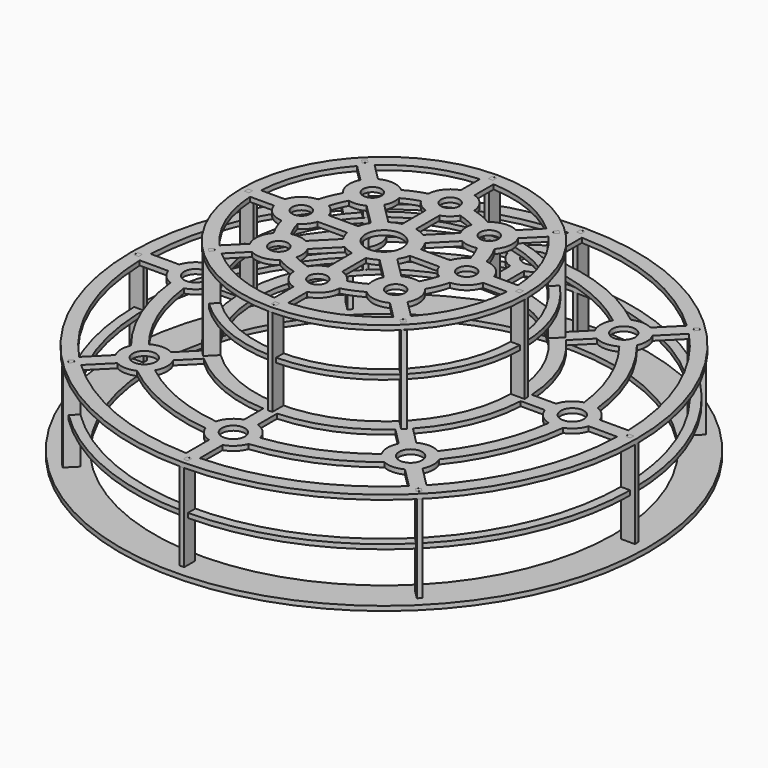
from build123d import *

# Parameters (mm, degrees)
F4_R      = 550
F4_R_2    = 25
F4_R_3    = 280
F5_DEPTH  = 10
F6_R      = 310
F6_R_2    = 20
F6_R_3    = 40
F7_DEPTH  = 10
F8_R      = 575
F8_R_2    = 500
F9_DEPTH  = 10
F11_DEPTH = 5
F12_COUNT = 8
F13_R     = 520
F14_DEPTH = 10
F15_R     = 280
F16_DEPTH = 10


with BuildPart() as f5:
    # F4 (on Top) → F5 (new body)
    with BuildSketch(Plane.XY):
        Circle(F4_R)
        Polygon((-374.0594872477, -375.4737008101), (-371.3017708011, -378.2314172567), (-378.3728386129, -385.3024850685), (-381.1305550595, -382.5447686219), (-382.5447686219, -382.5447686219), (-382.5447686219, -381.1305550595), (-385.3024850685, -378.3728386129), (-378.2314172567, -371.3017708011), (-375.4737008101, -374.0594872477), (-374.0594872477, -374.0594872477), align=None, mode=Mode.SUBTRACT)
        with Locations((-289.9137802865, -289.9137802865)):
            Circle(F4_R_2, mode=Mode.SUBTRACT)
        with BuildLine():
            ThreePointArc((-46.8602222393, -427.4390243902), (-34.4319247471, -446.2552418033), (-15, -457.6969600708))
            Line((-15, -457.6969600708), (-15, -519.783608822))
            ThreePointArc((-15, -519.783608822), (-198.9953848298, -480.4173569059), (-356.9359128298, -378.1491162654))
            Line((-356.9359128298, -378.1491162654), (-313.0340224768, -334.2472259124))
            ThreePointArc((-313.0340224768, -334.2472259124), (-291.2030601412, -339.8971550971), (-269.1098517768, -335.3802136034))
            ThreePointArc((-269.1098517768, -335.3802136034), (-164.553875917, -397.2681989799), (-46.8602222393, -427.4390243902))
        make_face(mode=Mode.SUBTRACT)
        with BuildLine():
            Line((-15, -309.6368841078), (-15, -362.3030399292))
            ThreePointArc((-15, -362.3030399292), (-36.1104599854, -375.4162656782), (-48.3000733443, -397.0731707317))
            ThreePointArc((-48.3000733443, -397.0731707317), (-153.073372946, -369.5518130045), (-246.619822258, -314.9264410452))
            ThreePointArc((-246.619822258, -314.9264410452), (-239.9254361013, -290.9933383562), (-245.5803346606, -266.7935380962))
            Line((-245.5803346606, -266.7935380962), (-208.3397387403, -229.5529421759))
            ThreePointArc((-208.3397387403, -229.5529421759), (-118.6318640332, -286.4026550785), (-15, -309.6368841078))
        make_face(mode=Mode.SUBTRACT)
        with BuildLine():
            Line((-519.783608822, -15), (-457.6969600708, -15))
            ThreePointArc((-457.6969600708, -15), (-446.2552418033, -34.4319247471), (-427.4390243902, -46.8602222393))
            ThreePointArc((-427.4390243902, -46.8602222393), (-397.2681989799, -164.553875917), (-335.3802136034, -269.1098517768))
            ThreePointArc((-335.3802136034, -269.1098517768), (-339.8971550971, -291.2030601412), (-334.2472259124, -313.0340224768))
            Line((-334.2472259124, -313.0340224768), (-378.1491162654, -356.9359128298))
            ThreePointArc((-378.1491162654, -356.9359128298), (-480.4173569059, -198.9953848298), (-519.783608822, -15))
        make_face(mode=Mode.SUBTRACT)
        with BuildLine():
            ThreePointArc((-397.0731707317, -48.3000733443), (-375.4162656782, -36.1104599854), (-362.3030399292, -15))
            Line((-362.3030399292, -15), (-309.6368841078, -15))
            ThreePointArc((-309.6368841078, -15), (-286.4026550785, -118.6318640332), (-229.5529421759, -208.3397387403))
            Line((-229.5529421759, -208.3397387403), (-266.7935380962, -245.5803346606))
            ThreePointArc((-266.7935380962, -245.5803346606), (-290.9933383562, -239.9254361013), (-314.9264410452, -246.619822258))
            ThreePointArc((-314.9264410452, -246.619822258), (-369.5518130045, -153.073372946), (-397.0731707317, -48.3000733443))
        make_face(mode=Mode.SUBTRACT)
        Polygon((-215.5968575838, -208.6672111282), (-208.5257897719, -201.5961433163), (-205.7680733253, -204.3538597629), (-204.3538597629, -204.3538597629), (-204.3538597629, -205.7680733253), (-201.5961433163, -208.5257897719), (-208.6672111282, -215.5968575838), (-211.4249275748, -212.8391411372), (-212.8391411372, -212.8391411372), (-212.8391411372, -211.4249275748), align=None, mode=Mode.SUBTRACT)
        Polygon((1, -530), (4.9, -530), (4.9, -540), (1, -540), (0, -541), (-1, -540), (-4.9, -540), (-4.9, -530), (-1, -530), (0, -529), align=None, mode=Mode.SUBTRACT)
        with BuildLine():
            ThreePointArc((356.9359128298, -378.1491162654), (198.9953848298, -480.4173569059), (15, -519.783608822))
            Line((15, -519.783608822), (15, -457.6969600708))
            ThreePointArc((15, -457.6969600708), (34.4319247471, -446.2552418033), (46.8602222393, -427.4390243902))
            ThreePointArc((46.8602222393, -427.4390243902), (164.553875917, -397.2681989799), (269.1098517768, -335.3802136034))
            ThreePointArc((269.1098517768, -335.3802136034), (291.2030601412, -339.8971550971), (313.0340224768, -334.2472259124))
            Line((313.0340224768, -334.2472259124), (356.9359128298, -378.1491162654))
        make_face(mode=Mode.SUBTRACT)
        with Locations((0, -410)):
            Circle(F4_R_2, mode=Mode.SUBTRACT)
        Polygon((-4.9, -300), (-4.9, -290), (-1, -290), (0, -289), (1, -290), (4.9, -290), (4.9, -300), (1, -300), (0, -301), (-1, -300), align=None, mode=Mode.SUBTRACT)
        with BuildLine():
            ThreePointArc((246.619822258, -314.9264410452), (153.073372946, -369.5518130045), (48.3000733443, -397.0731707317))
            ThreePointArc((48.3000733443, -397.0731707317), (36.1104599854, -375.4162656782), (15, -362.3030399292))
            Line((15, -362.3030399292), (15, -309.6368841078))
            ThreePointArc((15, -309.6368841078), (118.6318640332, -286.4026550785), (208.3397387403, -229.5529421759))
            Line((208.3397387403, -229.5529421759), (245.5803346606, -266.7935380962))
            ThreePointArc((245.5803346606, -266.7935380962), (239.9254361013, -290.9933383562), (246.619822258, -314.9264410452))
        make_face(mode=Mode.SUBTRACT)
        Polygon((375.4737008101, -374.0594872477), (378.2314172567, -371.3017708011), (385.3024850685, -378.3728386129), (382.5447686219, -381.1305550595), (382.5447686219, -382.5447686219), (381.1305550595, -382.5447686219), (378.3728386129, -385.3024850685), (371.3017708011, -378.2314172567), (374.0594872477, -375.4737008101), (374.0594872477, -374.0594872477), align=None, mode=Mode.SUBTRACT)
        with Locations((289.9137802865, -289.9137802865)):
            Circle(F4_R_2, mode=Mode.SUBTRACT)
        Polygon((208.6672111282, -215.5968575838), (201.5961433163, -208.5257897719), (204.3538597629, -205.7680733253), (204.3538597629, -204.3538597629), (205.7680733253, -204.3538597629), (208.5257897719, -201.5961433163), (215.5968575838, -208.6672111282), (212.8391411372, -211.4249275748), (212.8391411372, -212.8391411372), (211.4249275748, -212.8391411372), align=None, mode=Mode.SUBTRACT)
        with BuildLine():
            Line((378.1491162654, -356.9359128298), (334.2472259124, -313.0340224768))
            ThreePointArc((334.2472259124, -313.0340224768), (339.8971550971, -291.2030601412), (335.3802136034, -269.1098517768))
            ThreePointArc((335.3802136034, -269.1098517768), (397.2681989799, -164.553875917), (427.4390243902, -46.8602222393))
            ThreePointArc((427.4390243902, -46.8602222393), (446.2552418033, -34.4319247471), (457.6969600708, -15))
            Line((457.6969600708, -15), (519.783608822, -15))
            ThreePointArc((519.783608822, -15), (480.4173569059, -198.9953848298), (378.1491162654, -356.9359128298))
        make_face(mode=Mode.SUBTRACT)
        with BuildLine():
            ThreePointArc((314.9264410452, -246.619822258), (290.9933383562, -239.9254361013), (266.7935380962, -245.5803346606))
            Line((266.7935380962, -245.5803346606), (229.5529421759, -208.3397387403))
            ThreePointArc((229.5529421759, -208.3397387403), (286.4026550785, -118.6318640332), (309.6368841078, -15))
            Line((309.6368841078, -15), (362.3030399292, -15))
            ThreePointArc((362.3030399292, -15), (375.4162656782, -36.1104599854), (397.0731707317, -48.3000733443))
            ThreePointArc((397.0731707317, -48.3000733443), (369.5518130045, -153.073372946), (314.9264410452, -246.619822258))
        make_face(mode=Mode.SUBTRACT)
        Polygon((-530, -1), (-530, -4.9), (-540, -4.9), (-540, -1), (-541, 0), (-540, 1), (-540, 4.9), (-530, 4.9), (-530, 1), (-529, 0), align=None, mode=Mode.SUBTRACT)
        with Locations((-410, 0)):
            Circle(F4_R_2, mode=Mode.SUBTRACT)
        Polygon((-300, 4.9), (-290, 4.9), (-290, 1), (-289, 0), (-290, -1), (-290, -4.9), (-300, -4.9), (-300, -1), (-301, 0), (-300, 1), align=None, mode=Mode.SUBTRACT)
        with BuildLine():
            ThreePointArc((-314.9264410452, 246.619822258), (-290.9933383562, 239.9254361013), (-266.7935380962, 245.5803346606))
            Line((-266.7935380962, 245.5803346606), (-229.5529421759, 208.3397387403))
            ThreePointArc((-229.5529421759, 208.3397387403), (-286.4026550785, 118.6318640332), (-309.6368841078, 15))
            Line((-309.6368841078, 15), (-362.3030399292, 15))
            ThreePointArc((-362.3030399292, 15), (-375.4162656782, 36.1104599854), (-397.0731707317, 48.3000733443))
            ThreePointArc((-397.0731707317, 48.3000733443), (-369.5518130045, 153.073372946), (-314.9264410452, 246.619822258))
        make_face(mode=Mode.SUBTRACT)
        with BuildLine():
            Line((-378.1491162654, 356.9359128298), (-334.2472259124, 313.0340224768))
            ThreePointArc((-334.2472259124, 313.0340224768), (-339.8971550971, 291.2030601412), (-335.3802136034, 269.1098517768))
            ThreePointArc((-335.3802136034, 269.1098517768), (-397.2681989799, 164.553875917), (-427.4390243902, 46.8602222393))
            ThreePointArc((-427.4390243902, 46.8602222393), (-446.2552418033, 34.4319247471), (-457.6969600708, 15))
            Line((-457.6969600708, 15), (-519.783608822, 15))
            ThreePointArc((-519.783608822, 15), (-480.4173569059, 198.9953848298), (-378.1491162654, 356.9359128298))
        make_face(mode=Mode.SUBTRACT)
        Polygon((-208.6672111282, 215.5968575838), (-201.5961433163, 208.5257897719), (-204.3538597629, 205.7680733253), (-204.3538597629, 204.3538597629), (-205.7680733253, 204.3538597629), (-208.5257897719, 201.5961433163), (-215.5968575838, 208.6672111282), (-212.8391411372, 211.4249275748), (-212.8391411372, 212.8391411372), (-211.4249275748, 212.8391411372), align=None, mode=Mode.SUBTRACT)
        with Locations((-289.9137802865, 289.9137802865)):
            Circle(F4_R_2, mode=Mode.SUBTRACT)
        Polygon((-375.4737008101, 374.0594872477), (-378.2314172567, 371.3017708011), (-385.3024850685, 378.3728386129), (-382.5447686219, 381.1305550595), (-382.5447686219, 382.5447686219), (-381.1305550595, 382.5447686219), (-378.3728386129, 385.3024850685), (-371.3017708011, 378.2314172567), (-374.0594872477, 375.4737008101), (-374.0594872477, 374.0594872477), align=None, mode=Mode.SUBTRACT)
        with BuildLine():
            ThreePointArc((-48.3000733443, 397.0731707317), (-36.1104599854, 375.4162656782), (-15, 362.3030399292))
            Line((-15, 362.3030399292), (-15, 309.6368841078))
            ThreePointArc((-15, 309.6368841078), (-118.6318640332, 286.4026550785), (-208.3397387403, 229.5529421759))
            Line((-208.3397387403, 229.5529421759), (-245.5803346606, 266.7935380962))
            ThreePointArc((-245.5803346606, 266.7935380962), (-239.9254361013, 290.9933383562), (-246.619822258, 314.9264410452))
            ThreePointArc((-246.619822258, 314.9264410452), (-153.073372946, 369.5518130045), (-48.3000733443, 397.0731707317))
        make_face(mode=Mode.SUBTRACT)
        with BuildLine():
            Line((-15, 519.783608822), (-15, 457.6969600708))
            ThreePointArc((-15, 457.6969600708), (-34.4319247471, 446.2552418033), (-46.8602222393, 427.4390243902))
            ThreePointArc((-46.8602222393, 427.4390243902), (-164.553875917, 397.2681989799), (-269.1098517768, 335.3802136034))
            ThreePointArc((-269.1098517768, 335.3802136034), (-291.2030601412, 339.8971550971), (-313.0340224768, 334.2472259124))
            Line((-313.0340224768, 334.2472259124), (-356.9359128298, 378.1491162654))
            ThreePointArc((-356.9359128298, 378.1491162654), (-198.9953848298, 480.4173569059), (-15, 519.783608822))
        make_face(mode=Mode.SUBTRACT)
        Circle(F4_R_3, mode=Mode.SUBTRACT)
        Polygon((215.5968575838, 208.6672111282), (208.5257897719, 201.5961433163), (205.7680733253, 204.3538597629), (204.3538597629, 204.3538597629), (204.3538597629, 205.7680733253), (201.5961433163, 208.5257897719), (208.6672111282, 215.5968575838), (211.4249275748, 212.8391411372), (212.8391411372, 212.8391411372), (212.8391411372, 211.4249275748), align=None, mode=Mode.SUBTRACT)
        Polygon((300, -4.9), (290, -4.9), (290, -1), (289, 0), (290, 1), (290, 4.9), (300, 4.9), (300, 1), (301, 0), (300, -1), align=None, mode=Mode.SUBTRACT)
        with Locations((410, 0)):
            Circle(F4_R_2, mode=Mode.SUBTRACT)
        with BuildLine():
            ThreePointArc((397.0731707317, 48.3000733443), (375.4162656782, 36.1104599854), (362.3030399292, 15))
            Line((362.3030399292, 15), (309.6368841078, 15))
            ThreePointArc((309.6368841078, 15), (286.4026550785, 118.6318640332), (229.5529421759, 208.3397387403))
            Line((229.5529421759, 208.3397387403), (266.7935380962, 245.5803346606))
            ThreePointArc((266.7935380962, 245.5803346606), (290.9933383562, 239.9254361013), (314.9264410452, 246.619822258))
            ThreePointArc((314.9264410452, 246.619822258), (369.5518130045, 153.073372946), (397.0731707317, 48.3000733443))
        make_face(mode=Mode.SUBTRACT)
        Polygon((530, 1), (530, 4.9), (540, 4.9), (540, 1), (541, 0), (540, -1), (540, -4.9), (530, -4.9), (530, -1), (529, 0), align=None, mode=Mode.SUBTRACT)
        with BuildLine():
            Line((519.783608822, 15), (457.6969600708, 15))
            ThreePointArc((457.6969600708, 15), (446.2552418033, 34.4319247471), (427.4390243902, 46.8602222393))
            ThreePointArc((427.4390243902, 46.8602222393), (397.2681989799, 164.553875917), (335.3802136034, 269.1098517768))
            ThreePointArc((335.3802136034, 269.1098517768), (339.8971550971, 291.2030601412), (334.2472259124, 313.0340224768))
            Line((334.2472259124, 313.0340224768), (378.1491162654, 356.9359128298))
            ThreePointArc((378.1491162654, 356.9359128298), (480.4173569059, 198.9953848298), (519.783608822, 15))
        make_face(mode=Mode.SUBTRACT)
        Polygon((4.9, 300), (4.9, 290), (1, 290), (0, 289), (-1, 290), (-4.9, 290), (-4.9, 300), (-1, 300), (0, 301), (1, 300), align=None, mode=Mode.SUBTRACT)
        with BuildLine():
            ThreePointArc((246.619822258, 314.9264410452), (239.9254361013, 290.9933383562), (245.5803346606, 266.7935380962))
            Line((245.5803346606, 266.7935380962), (208.3397387403, 229.5529421759))
            ThreePointArc((208.3397387403, 229.5529421759), (118.6318640332, 286.4026550785), (15, 309.6368841078))
            Line((15, 309.6368841078), (15, 362.3030399292))
            ThreePointArc((15, 362.3030399292), (36.1104599854, 375.4162656782), (48.3000733443, 397.0731707317))
            ThreePointArc((48.3000733443, 397.0731707317), (153.073372946, 369.5518130045), (246.619822258, 314.9264410452))
        make_face(mode=Mode.SUBTRACT)
        with Locations((0, 410)):
            Circle(F4_R_2, mode=Mode.SUBTRACT)
        Polygon((4.9, 540), (4.9, 530), (1, 530), (0, 529), (-1, 530), (-4.9, 530), (-4.9, 540), (-1, 540), (0, 541), (1, 540), align=None, mode=Mode.SUBTRACT)
        with BuildLine():
            Line((356.9359128298, 378.1491162654), (313.0340224768, 334.2472259124))
            ThreePointArc((313.0340224768, 334.2472259124), (291.2030601412, 339.8971550971), (269.1098517768, 335.3802136034))
            ThreePointArc((269.1098517768, 335.3802136034), (164.553875917, 397.2681989799), (46.8602222393, 427.4390243902))
            ThreePointArc((46.8602222393, 427.4390243902), (34.4319247471, 446.2552418033), (15, 457.6969600708))
            Line((15, 457.6969600708), (15, 519.783608822))
            ThreePointArc((15, 519.783608822), (198.9953848298, 480.4173569059), (356.9359128298, 378.1491162654))
        make_face(mode=Mode.SUBTRACT)
        with Locations((289.9137802865, 289.9137802865)):
            Circle(F4_R_2, mode=Mode.SUBTRACT)
        Polygon((374.0594872477, 375.4737008101), (371.3017708011, 378.2314172567), (378.3728386129, 385.3024850685), (381.1305550595, 382.5447686219), (382.5447686219, 382.5447686219), (382.5447686219, 381.1305550595), (385.3024850685, 378.3728386129), (378.2314172567, 371.3017708011), (375.4737008101, 374.0594872477), (374.0594872477, 374.0594872477), align=None, mode=Mode.SUBTRACT)
    extrude(amount=F5_DEPTH)


with BuildPart() as f7:
    # F6 (on offset) → F7 (new body)
    with BuildSketch(Plane.XY.offset(200)):
        Circle(F6_R)
        Polygon((-204.3538597629, -204.3538597629), (-204.3538597629, -205.7680733253), (-201.5961433163, -208.5257897719), (-208.6672111282, -215.5968575838), (-211.4249275748, -212.8391411372), (-212.8391411372, -212.8391411372), (-212.8391411372, -211.4249275748), (-215.5968575838, -208.6672111282), (-208.5257897719, -201.5961433163), (-205.7680733253, -204.3538597629), align=None, mode=Mode.SUBTRACT)
        with BuildLine():
            ThreePointArc((-49.888765157, -183.3333333333), (-39.3023002536, -210.9084000682), (-15, -227.6969600708))
            Line((-15, -227.6969600708), (-15, -279.5979256003))
            ThreePointArc((-15, -279.5979256003), (-107.1513610622, -258.6862691032), (-187.0989874799, -208.3121909155))
            Line((-187.0989874799, -208.3121909155), (-150.3994628039, -171.6126662395))
            ThreePointArc((-150.3994628039, -171.6126662395), (-121.3438368718, -176.925682923), (-94.35955907, -164.9129273651))
            ThreePointArc((-94.35955907, -164.9129273651), (-72.7098521494, -175.5371111771), (-49.888765157, -183.3333333333))
        make_face(mode=Mode.SUBTRACT)
        with BuildLine():
            Line((-279.5979256003, -15), (-227.6969600708, -15))
            ThreePointArc((-227.6969600708, -15), (-210.9084000682, -39.3023002536), (-183.3333333333, -49.888765157))
            ThreePointArc((-183.3333333333, -49.888765157), (-175.5371111771, -72.7098521494), (-164.9129273651, -94.35955907))
            ThreePointArc((-164.9129273651, -94.35955907), (-176.925682923, -121.3438368718), (-171.6126662395, -150.3994628039))
            Line((-171.6126662395, -150.3994628039), (-208.3121909155, -187.0989874799))
            ThreePointArc((-208.3121909155, -187.0989874799), (-258.6862691032, -107.1513610622), (-279.5979256003, -15))
        make_face(mode=Mode.SUBTRACT)
        with Locations((-127.2792206136, -127.2792206136)):
            Circle(F6_R_2, mode=Mode.SUBTRACT)
        with BuildLine():
            Line((-15, -68.3739716559), (-15, -132.3030399292))
            ThreePointArc((-15, -132.3030399292), (-30.9028195191, -140.6933116916), (-42.8093317968, -154.1666666667))
            ThreePointArc((-42.8093317968, -154.1666666667), (-61.2293491784, -147.8207252018), (-78.7415266213, -139.2830642445))
            ThreePointArc((-78.7415266213, -139.2830642445), (-77.633601525, -121.3367880044), (-82.9457749877, -104.1589784233))
            Line((-82.9457749877, -104.1589784233), (-37.7410972967, -58.9543007323))
            ThreePointArc((-37.7410972967, -58.9543007323), (-26.7878402656, -64.6715672758), (-15, -68.3739716559))
        make_face(mode=Mode.SUBTRACT)
        with BuildLine():
            Line((-132.3030399292, -15), (-68.3739716559, -15))
            ThreePointArc((-68.3739716559, -15), (-64.6715672758, -26.7878402656), (-58.9543007323, -37.7410972967))
            Line((-58.9543007323, -37.7410972967), (-104.1589784233, -82.9457749877))
            ThreePointArc((-104.1589784233, -82.9457749877), (-121.3367880044, -77.633601525), (-139.2830642445, -78.7415266213))
            ThreePointArc((-139.2830642445, -78.7415266213), (-147.8207252018, -61.2293491784), (-154.1666666667, -42.8093317968))
            ThreePointArc((-154.1666666667, -42.8093317968), (-140.6933116916, -30.9028195191), (-132.3030399292, -15))
        make_face(mode=Mode.SUBTRACT)
        Polygon((0, -289), (1, -290), (4.9, -290), (4.9, -300), (1, -300), (0, -301), (-1, -300), (-4.9, -300), (-4.9, -290), (-1, -290), align=None, mode=Mode.SUBTRACT)
        with Locations((0, -180)):
            Circle(F6_R_2, mode=Mode.SUBTRACT)
        with BuildLine():
            ThreePointArc((15, -227.6969600708), (39.3023002536, -210.9084000682), (49.888765157, -183.3333333333))
            ThreePointArc((49.888765157, -183.3333333333), (72.7098521494, -175.5371111771), (94.35955907, -164.9129273651))
            ThreePointArc((94.35955907, -164.9129273651), (121.3438368718, -176.925682923), (150.3994628039, -171.6126662395))
            Line((150.3994628039, -171.6126662395), (187.0989874799, -208.3121909155))
            ThreePointArc((187.0989874799, -208.3121909155), (107.1513610622, -258.6862691032), (15, -279.5979256003))
            Line((15, -279.5979256003), (15, -227.6969600708))
        make_face(mode=Mode.SUBTRACT)
        Polygon((204.3538597629, -204.3538597629), (205.7680733253, -204.3538597629), (208.5257897719, -201.5961433163), (215.5968575838, -208.6672111282), (212.8391411372, -211.4249275748), (212.8391411372, -212.8391411372), (211.4249275748, -212.8391411372), (208.6672111282, -215.5968575838), (201.5961433163, -208.5257897719), (204.3538597629, -205.7680733253), align=None, mode=Mode.SUBTRACT)
        with BuildLine():
            ThreePointArc((78.7415266213, -139.2830642445), (61.2293491784, -147.8207252018), (42.8093317968, -154.1666666667))
            ThreePointArc((42.8093317968, -154.1666666667), (30.9028195191, -140.6933116916), (15, -132.3030399292))
            Line((15, -132.3030399292), (15, -68.3739716559))
            ThreePointArc((15, -68.3739716559), (26.7878402656, -64.6715672758), (37.7410972967, -58.9543007323))
            Line((37.7410972967, -58.9543007323), (82.9457749877, -104.1589784233))
            ThreePointArc((82.9457749877, -104.1589784233), (77.633601525, -121.3367880044), (78.7415266213, -139.2830642445))
        make_face(mode=Mode.SUBTRACT)
        with Locations((127.2792206136, -127.2792206136)):
            Circle(F6_R_2, mode=Mode.SUBTRACT)
        with BuildLine():
            Line((104.1589784233, -82.9457749877), (58.9543007323, -37.7410972967))
            ThreePointArc((58.9543007323, -37.7410972967), (64.6715672758, -26.7878402656), (68.3739716559, -15))
            Line((68.3739716559, -15), (132.3030399292, -15))
            ThreePointArc((132.3030399292, -15), (140.6933116916, -30.9028195191), (154.1666666667, -42.8093317968))
            ThreePointArc((154.1666666667, -42.8093317968), (147.8207252018, -61.2293491784), (139.2830642445, -78.7415266213))
            ThreePointArc((139.2830642445, -78.7415266213), (121.3367880044, -77.633601525), (104.1589784233, -82.9457749877))
        make_face(mode=Mode.SUBTRACT)
        with BuildLine():
            Line((208.3121909155, -187.0989874799), (171.6126662395, -150.3994628039))
            ThreePointArc((171.6126662395, -150.3994628039), (176.925682923, -121.3438368718), (164.9129273651, -94.35955907))
            ThreePointArc((164.9129273651, -94.35955907), (175.5371111771, -72.7098521494), (183.3333333333, -49.888765157))
            ThreePointArc((183.3333333333, -49.888765157), (210.9084000682, -39.3023002536), (227.6969600708, -15))
            Line((227.6969600708, -15), (279.5979256003, -15))
            ThreePointArc((279.5979256003, -15), (258.6862691032, -107.1513610622), (208.3121909155, -187.0989874799))
        make_face(mode=Mode.SUBTRACT)
        Polygon((-289, 0), (-290, -1), (-290, -4.9), (-300, -4.9), (-300, -1), (-301, 0), (-300, 1), (-300, 4.9), (-290, 4.9), (-290, 1), align=None, mode=Mode.SUBTRACT)
        with Locations((-180, 0)):
            Circle(F6_R_2, mode=Mode.SUBTRACT)
        with BuildLine():
            Line((-208.3121909155, 187.0989874799), (-171.6126662395, 150.3994628039))
            ThreePointArc((-171.6126662395, 150.3994628039), (-176.925682923, 121.3438368718), (-164.9129273651, 94.35955907))
            ThreePointArc((-164.9129273651, 94.35955907), (-175.5371111771, 72.7098521494), (-183.3333333333, 49.888765157))
            ThreePointArc((-183.3333333333, 49.888765157), (-210.9084000682, 39.3023002536), (-227.6969600708, 15))
            Line((-227.6969600708, 15), (-279.5979256003, 15))
            ThreePointArc((-279.5979256003, 15), (-258.6862691032, 107.1513610622), (-208.3121909155, 187.0989874799))
        make_face(mode=Mode.SUBTRACT)
        with BuildLine():
            Line((-104.1589784233, 82.9457749877), (-58.9543007323, 37.7410972967))
            ThreePointArc((-58.9543007323, 37.7410972967), (-64.6715672758, 26.7878402656), (-68.3739716559, 15))
            Line((-68.3739716559, 15), (-132.3030399292, 15))
            ThreePointArc((-132.3030399292, 15), (-140.6933116916, 30.9028195191), (-154.1666666667, 42.8093317968))
            ThreePointArc((-154.1666666667, 42.8093317968), (-147.8207252018, 61.2293491784), (-139.2830642445, 78.7415266213))
            ThreePointArc((-139.2830642445, 78.7415266213), (-121.3367880044, 77.633601525), (-104.1589784233, 82.9457749877))
        make_face(mode=Mode.SUBTRACT)
        with Locations((-127.2792206136, 127.2792206136)):
            Circle(F6_R_2, mode=Mode.SUBTRACT)
        with BuildLine():
            Line((-15, 132.3030399292), (-15, 68.3739716559))
            ThreePointArc((-15, 68.3739716559), (-26.7878402656, 64.6715672758), (-37.7410972967, 58.9543007323))
            Line((-37.7410972967, 58.9543007323), (-82.9457749877, 104.1589784233))
            ThreePointArc((-82.9457749877, 104.1589784233), (-77.633601525, 121.3367880044), (-78.7415266213, 139.2830642445))
            ThreePointArc((-78.7415266213, 139.2830642445), (-61.2293491784, 147.8207252018), (-42.8093317968, 154.1666666667))
            ThreePointArc((-42.8093317968, 154.1666666667), (-30.9028195191, 140.6933116916), (-15, 132.3030399292))
        make_face(mode=Mode.SUBTRACT)
        Polygon((-204.3538597629, 204.3538597629), (-205.7680733253, 204.3538597629), (-208.5257897719, 201.5961433163), (-215.5968575838, 208.6672111282), (-212.8391411372, 211.4249275748), (-212.8391411372, 212.8391411372), (-211.4249275748, 212.8391411372), (-208.6672111282, 215.5968575838), (-201.5961433163, 208.5257897719), (-204.3538597629, 205.7680733253), align=None, mode=Mode.SUBTRACT)
        with BuildLine():
            Line((-15, 279.5979256003), (-15, 227.6969600708))
            ThreePointArc((-15, 227.6969600708), (-39.3023002536, 210.9084000682), (-49.888765157, 183.3333333333))
            ThreePointArc((-49.888765157, 183.3333333333), (-72.7098521494, 175.5371111771), (-94.35955907, 164.9129273651))
            ThreePointArc((-94.35955907, 164.9129273651), (-121.3438368718, 176.925682923), (-150.3994628039, 171.6126662395))
            Line((-150.3994628039, 171.6126662395), (-187.0989874799, 208.3121909155))
            ThreePointArc((-187.0989874799, 208.3121909155), (-107.1513610622, 258.6862691032), (-15, 279.5979256003))
        make_face(mode=Mode.SUBTRACT)
        Circle(F6_R_3, mode=Mode.SUBTRACT)
        with BuildLine():
            Line((132.3030399292, 15), (68.3739716559, 15))
            ThreePointArc((68.3739716559, 15), (64.6715672758, 26.7878402656), (58.9543007323, 37.7410972967))
            Line((58.9543007323, 37.7410972967), (104.1589784233, 82.9457749877))
            ThreePointArc((104.1589784233, 82.9457749877), (121.3367880044, 77.633601525), (139.2830642445, 78.7415266213))
            ThreePointArc((139.2830642445, 78.7415266213), (147.8207252018, 61.2293491784), (154.1666666667, 42.8093317968))
            ThreePointArc((154.1666666667, 42.8093317968), (140.6933116916, 30.9028195191), (132.3030399292, 15))
        make_face(mode=Mode.SUBTRACT)
        with BuildLine():
            Line((82.9457749877, 104.1589784233), (37.7410972967, 58.9543007323))
            ThreePointArc((37.7410972967, 58.9543007323), (26.7878402656, 64.6715672758), (15, 68.3739716559))
            Line((15, 68.3739716559), (15, 132.3030399292))
            ThreePointArc((15, 132.3030399292), (30.9028195191, 140.6933116916), (42.8093317968, 154.1666666667))
            ThreePointArc((42.8093317968, 154.1666666667), (61.2293491784, 147.8207252018), (78.7415266213, 139.2830642445))
            ThreePointArc((78.7415266213, 139.2830642445), (77.633601525, 121.3367880044), (82.9457749877, 104.1589784233))
        make_face(mode=Mode.SUBTRACT)
        with Locations((127.2792206136, 127.2792206136)):
            Circle(F6_R_2, mode=Mode.SUBTRACT)
        with Locations((180, 0)):
            Circle(F6_R_2, mode=Mode.SUBTRACT)
        Polygon((289, 0), (290, 1), (290, 4.9), (300, 4.9), (300, 1), (301, 0), (300, -1), (300, -4.9), (290, -4.9), (290, -1), align=None, mode=Mode.SUBTRACT)
        with BuildLine():
            Line((279.5979256003, 15), (227.6969600708, 15))
            ThreePointArc((227.6969600708, 15), (210.9084000682, 39.3023002536), (183.3333333333, 49.888765157))
            ThreePointArc((183.3333333333, 49.888765157), (175.5371111771, 72.7098521494), (164.9129273651, 94.35955907))
            ThreePointArc((164.9129273651, 94.35955907), (176.925682923, 121.3438368718), (171.6126662395, 150.3994628039))
            Line((171.6126662395, 150.3994628039), (208.3121909155, 187.0989874799))
            ThreePointArc((208.3121909155, 187.0989874799), (258.6862691032, 107.1513610622), (279.5979256003, 15))
        make_face(mode=Mode.SUBTRACT)
        with Locations((0, 180)):
            Circle(F6_R_2, mode=Mode.SUBTRACT)
        with BuildLine():
            Line((187.0989874799, 208.3121909155), (150.3994628039, 171.6126662395))
            ThreePointArc((150.3994628039, 171.6126662395), (121.3438368718, 176.925682923), (94.35955907, 164.9129273651))
            ThreePointArc((94.35955907, 164.9129273651), (72.7098521494, 175.5371111771), (49.888765157, 183.3333333333))
            ThreePointArc((49.888765157, 183.3333333333), (39.3023002536, 210.9084000682), (15, 227.6969600708))
            Line((15, 227.6969600708), (15, 279.5979256003))
            ThreePointArc((15, 279.5979256003), (107.1513610622, 258.6862691032), (187.0989874799, 208.3121909155))
        make_face(mode=Mode.SUBTRACT)
        Polygon((-1, 290), (-4.9, 290), (-4.9, 300), (-1, 300), (0, 301), (1, 300), (4.9, 300), (4.9, 290), (1, 290), (0, 289), align=None, mode=Mode.SUBTRACT)
        Polygon((204.3538597629, 204.3538597629), (204.3538597629, 205.7680733253), (201.5961433163, 208.5257897719), (208.6672111282, 215.5968575838), (211.4249275748, 212.8391411372), (212.8391411372, 212.8391411372), (212.8391411372, 211.4249275748), (215.5968575838, 208.6672111282), (208.5257897719, 201.5961433163), (205.7680733253, 204.3538597629), align=None, mode=Mode.SUBTRACT)
    extrude(amount=F7_DEPTH)


with BuildPart() as f9:
    # F8 (on offset) → F9 (new body)
    with BuildSketch(Plane.XY.offset(-200)):
        Circle(F8_R)
        Polygon((-374.0594872477, -375.4737008101), (-371.3017708011, -378.2314172567), (-378.3728386129, -385.3024850685), (-381.1305550595, -382.5447686219), (-382.5447686219, -382.5447686219), (-382.5447686219, -381.1305550595), (-385.3024850685, -378.3728386129), (-378.2314172567, -371.3017708011), (-375.4737008101, -374.0594872477), (-374.0594872477, -374.0594872477), align=None, mode=Mode.SUBTRACT)
        Polygon((1, -530), (4.9, -530), (4.9, -540), (1, -540), (0, -541), (-1, -540), (-4.9, -540), (-4.9, -530), (-1, -530), (0, -529), align=None, mode=Mode.SUBTRACT)
        Polygon((375.4737008101, -374.0594872477), (378.2314172567, -371.3017708011), (385.3024850685, -378.3728386129), (382.5447686219, -381.1305550595), (382.5447686219, -382.5447686219), (381.1305550595, -382.5447686219), (378.3728386129, -385.3024850685), (371.3017708011, -378.2314172567), (374.0594872477, -375.4737008101), (374.0594872477, -374.0594872477), align=None, mode=Mode.SUBTRACT)
        Polygon((-530, -1), (-530, -4.9), (-540, -4.9), (-540, -1), (-541, 0), (-540, 1), (-540, 4.9), (-530, 4.9), (-530, 1), (-529, 0), align=None, mode=Mode.SUBTRACT)
        Polygon((-375.4737008101, 374.0594872477), (-378.2314172567, 371.3017708011), (-385.3024850685, 378.3728386129), (-382.5447686219, 381.1305550595), (-382.5447686219, 382.5447686219), (-381.1305550595, 382.5447686219), (-378.3728386129, 385.3024850685), (-371.3017708011, 378.2314172567), (-374.0594872477, 375.4737008101), (-374.0594872477, 374.0594872477), align=None, mode=Mode.SUBTRACT)
        Circle(F8_R_2, mode=Mode.SUBTRACT)
        Polygon((530, 1), (530, 4.9), (540, 4.9), (540, 1), (541, 0), (540, -1), (540, -4.9), (530, -4.9), (530, -1), (529, 0), align=None, mode=Mode.SUBTRACT)
        Polygon((4.9, 540), (4.9, 530), (1, 530), (0, 529), (-1, 530), (-4.9, 530), (-4.9, 540), (-1, 540), (0, 541), (1, 540), align=None, mode=Mode.SUBTRACT)
        Polygon((374.0594872477, 375.4737008101), (371.3017708011, 378.2314172567), (378.3728386129, 385.3024850685), (381.1305550595, 382.5447686219), (382.5447686219, 382.5447686219), (382.5447686219, 381.1305550595), (385.3024850685, 378.3728386129), (378.2314172567, 371.3017708011), (375.4737008101, 374.0594872477), (374.0594872477, 374.0594872477), align=None, mode=Mode.SUBTRACT)
    extrude(amount=F9_DEPTH)


with BuildPart() as f11:
    # F10 (on Right) → F11 (new body, symmetric)
    with BuildSketch(Plane.YZ):
        Polygon((550, 0), (540, 0), (540, 10), (530, 10), (530, 0), (520, 0), (520, -90.1), (530, -90.1), (530, -99.9), (520, -99.9), (520, -190), (530, -190), (530, -200), (540, -200), (540, -190), (550, -190), align=None)
    extrude(amount=F11_DEPTH, both=True)


with BuildPart() as f11b:
    # F10 (on Right) → F11, piece 2 (new body, symmetric)
    with BuildSketch(Plane.YZ):
        Polygon((290, 10), (290, 0), (300, 0), (300, 10), (310, 10), (310, 200), (300, 200), (300, 210), (290, 210), (290, 200), (280, 200), (280, 109.9), (290, 109.9), (290, 100.1), (280, 100.1), (280, 10), align=None)
    extrude(amount=F11_DEPTH, both=True)


with BuildPart() as f12_1:
    # F12: instance of F11
    add(f11.part.rotate(Axis((0, 0, 210), (0, 0, 1)), 1 * 360 / F12_COUNT))


with BuildPart() as f12_2:
    # F12: instance of F11
    add(f11.part.rotate(Axis((0, 0, 210), (0, 0, 1)), 2 * 360 / F12_COUNT))


with BuildPart() as f12_3:
    # F12: instance of F11
    add(f11.part.rotate(Axis((0, 0, 210), (0, 0, 1)), 3 * 360 / F12_COUNT))


with BuildPart() as f12_4:
    # F12: instance of F11
    add(f11.part.rotate(Axis((0, 0, 210), (0, 0, 1)), 4 * 360 / F12_COUNT))


with BuildPart() as f12_5:
    # F12: instance of F11
    add(f11.part.rotate(Axis((0, 0, 210), (0, 0, 1)), 5 * 360 / F12_COUNT))


with BuildPart() as f12_6:
    # F12: instance of F11
    add(f11.part.rotate(Axis((0, 0, 210), (0, 0, 1)), 6 * 360 / F12_COUNT))


with BuildPart() as f12_7:
    # F12: instance of F11
    add(f11.part.rotate(Axis((0, 0, 210), (0, 0, 1)), 7 * 360 / F12_COUNT))


with BuildPart() as f12_8:
    # F12: instance of F11b
    add(f11b.part.rotate(Axis((0, 0, 210), (0, 0, 1)), 1 * 360 / F12_COUNT))


with BuildPart() as f12_9:
    # F12: instance of F11b
    add(f11b.part.rotate(Axis((0, 0, 210), (0, 0, 1)), 2 * 360 / F12_COUNT))


with BuildPart() as f12_10:
    # F12: instance of F11b
    add(f11b.part.rotate(Axis((0, 0, 210), (0, 0, 1)), 3 * 360 / F12_COUNT))


with BuildPart() as f12_11:
    # F12: instance of F11b
    add(f11b.part.rotate(Axis((0, 0, 210), (0, 0, 1)), 4 * 360 / F12_COUNT))


with BuildPart() as f12_12:
    # F12: instance of F11b
    add(f11b.part.rotate(Axis((0, 0, 210), (0, 0, 1)), 5 * 360 / F12_COUNT))


with BuildPart() as f12_13:
    # F12: instance of F11b
    add(f11b.part.rotate(Axis((0, 0, 210), (0, 0, 1)), 6 * 360 / F12_COUNT))


with BuildPart() as f12_14:
    # F12: instance of F11b
    add(f11b.part.rotate(Axis((0, 0, 210), (0, 0, 1)), 7 * 360 / F12_COUNT))


with BuildPart() as f14:
    # F13 (on offset) → F14 (new body)
    with BuildSketch(Plane.XY.offset(-100)):
        with BuildLine():
            Line((-530, -5), (-539.9768513557, -5))
            ThreePointArc((-539.9768513557, -5), (-498.8949475561, -206.6490534771), (-385.3568271833, -378.2857593714))
            Line((-385.3568271833, -378.2857593714), (-378.3021279348, -371.2310601229))
            Line((-378.3021279348, -371.2310601229), (-371.2310601229, -378.3021279348))
            Line((-371.2310601229, -378.3021279348), (-378.2857593714, -385.3568271833))
            ThreePointArc((-378.2857593714, -385.3568271833), (-206.6490534771, -498.8949475561), (-5, -539.9768513557))
            Line((-5, -539.9768513557), (-5, -530))
            Line((-5, -530), (5, -530))
            Line((5, -530), (5, -539.9768513557))
            ThreePointArc((5, -539.9768513557), (206.6490534771, -498.8949475561), (378.2857593714, -385.3568271833))
            Line((378.2857593714, -385.3568271833), (371.2310601229, -378.3021279348))
            Line((371.2310601229, -378.3021279348), (378.3021279348, -371.2310601229))
            Line((378.3021279348, -371.2310601229), (385.3568271833, -378.2857593714))
            ThreePointArc((385.3568271833, -378.2857593714), (498.8949475561, -206.6490534771), (539.9768513557, -5))
            Line((539.9768513557, -5), (530, -5))
            Line((530, -5), (530, 5))
            Line((530, 5), (539.9768513557, 5))
            ThreePointArc((539.9768513557, 5), (498.8949475561, 206.6490534771), (385.3568271833, 378.2857593714))
            Line((385.3568271833, 378.2857593714), (378.3021279348, 371.2310601229))
            Line((378.3021279348, 371.2310601229), (371.2310601229, 378.3021279348))
            Line((371.2310601229, 378.3021279348), (378.2857593714, 385.3568271833))
            ThreePointArc((378.2857593714, 385.3568271833), (206.6490534771, 498.8949475561), (5, 539.9768513557))
            Line((5, 539.9768513557), (5, 530))
            Line((5, 530), (-5, 530))
            Line((-5, 530), (-5, 539.9768513557))
            ThreePointArc((-5, 539.9768513557), (-206.6490534771, 498.8949475561), (-378.2857593714, 385.3568271833))
            Line((-378.2857593714, 385.3568271833), (-371.2310601229, 378.3021279348))
            Line((-371.2310601229, 378.3021279348), (-378.3021279348, 371.2310601229))
            Line((-378.3021279348, 371.2310601229), (-385.3568271833, 378.2857593714))
            ThreePointArc((-385.3568271833, 378.2857593714), (-498.8949475561, 206.6490534771), (-539.9768513557, 5))
            Line((-539.9768513557, 5), (-530, 5))
            Line((-530, 5), (-530, -5))
        make_face()
        Circle(F13_R, mode=Mode.SUBTRACT)
    extrude(amount=F14_DEPTH)


with BuildPart() as f16:
    # F15 (on offset) → F16 (new body)
    with BuildSketch(Plane.XY.offset(100)):
        with BuildLine():
            Line((-290, -5), (-299.9583304394, -5))
            ThreePointArc((-299.9583304394, -5), (-277.1638597534, -114.8050297095), (-215.638103433, -208.5670356212))
            Line((-215.638103433, -208.5670356212), (-208.59650045, -201.5254326382))
            Line((-208.59650045, -201.5254326382), (-201.5254326382, -208.59650045))
            Line((-201.5254326382, -208.59650045), (-208.5670356212, -215.638103433))
            ThreePointArc((-208.5670356212, -215.638103433), (-114.8050297095, -277.1638597534), (-5, -299.9583304394))
            Line((-5, -299.9583304394), (-5, -290))
            Line((-5, -290), (5, -290))
            Line((5, -290), (5, -299.9583304394))
            ThreePointArc((5, -299.9583304394), (114.8050297095, -277.1638597534), (208.5670356212, -215.638103433))
            Line((208.5670356212, -215.638103433), (201.5254326382, -208.59650045))
            Line((201.5254326382, -208.59650045), (208.59650045, -201.5254326382))
            Line((208.59650045, -201.5254326382), (215.638103433, -208.5670356212))
            ThreePointArc((215.638103433, -208.5670356212), (277.1638597534, -114.8050297095), (299.9583304394, -5))
            Line((299.9583304394, -5), (290, -5))
            Line((290, -5), (290, 5))
            Line((290, 5), (299.9583304394, 5))
            ThreePointArc((299.9583304394, 5), (277.1638597534, 114.8050297095), (215.638103433, 208.5670356212))
            Line((215.638103433, 208.5670356212), (208.59650045, 201.5254326382))
            Line((208.59650045, 201.5254326382), (201.5254326382, 208.59650045))
            Line((201.5254326382, 208.59650045), (208.5670356212, 215.638103433))
            ThreePointArc((208.5670356212, 215.638103433), (114.8050297095, 277.1638597534), (5, 299.9583304394))
            Line((5, 299.9583304394), (5, 290))
            Line((5, 290), (-5, 290))
            Line((-5, 290), (-5, 299.9583304394))
            ThreePointArc((-5, 299.9583304394), (-114.8050297095, 277.1638597534), (-208.5670356212, 215.638103433))
            Line((-208.5670356212, 215.638103433), (-201.5254326382, 208.59650045))
            Line((-201.5254326382, 208.59650045), (-208.59650045, 201.5254326382))
            Line((-208.59650045, 201.5254326382), (-215.638103433, 208.5670356212))
            ThreePointArc((-215.638103433, 208.5670356212), (-277.1638597534, 114.8050297095), (-299.9583304394, 5))
            Line((-299.9583304394, 5), (-290, 5))
            Line((-290, 5), (-290, -5))
        make_face()
        Circle(F15_R, mode=Mode.SUBTRACT)
    extrude(amount=F16_DEPTH)


solid = Compound([f5.part, f7.part, f9.part, f11.part, f11b.part, f12_1.part, f12_2.part, f12_3.part, f12_4.part, f12_5.part, f12_6.part, f12_7.part, f12_8.part, f12_9.part, f12_10.part, f12_11.part, f12_12.part, f12_13.part, f12_14.part, f14.part, f16.part])
